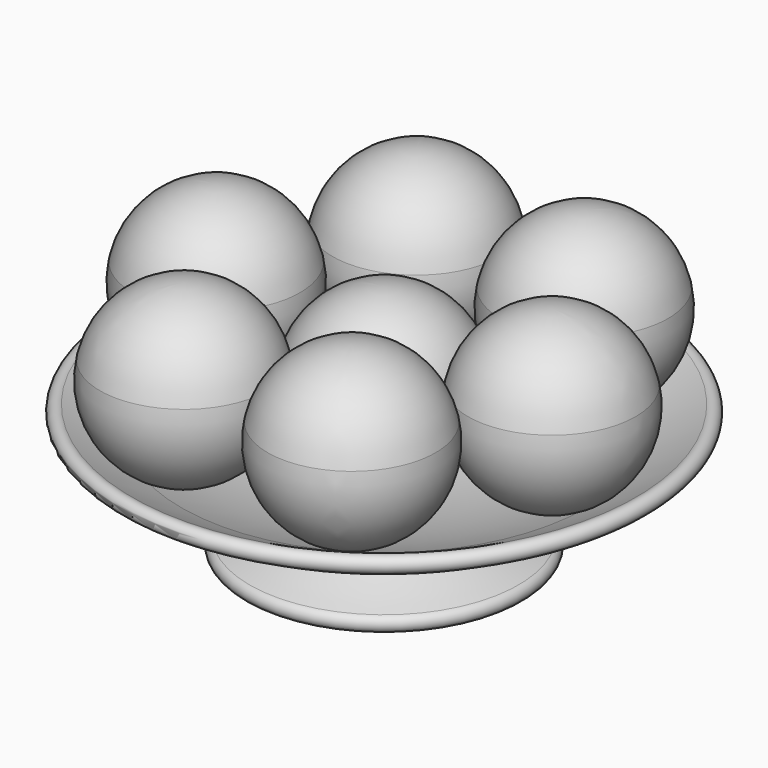
from build123d import *

# Parameters (mm, degrees)
F3_COUNT = 6


# Not quite as in the source:
# - ends of sketch curves that miss each other by under 0.0002 mm in the source are joined


with BuildPart() as f1:
    # F0 (on Front) → F1 (revolve)
    with BuildSketch(Plane.XZ):
        with BuildLine():
            Line((0, 0), (0, 6))
            ThreePointArc((0, 6), (-39.2492027787, 10.1203091704), (-76.7870949738, 22.3015864419))
            ThreePointArc((-76.7870949738, 22.3015864419), (-86.2691485264, 26.8374773841), (-95.484375, 31.8934883861))
            ThreePointArc((-95.484375, 31.8934883861), (-99.5889922478, 30.8201211382), (-98.515625, 26.7155038904))
            ThreePointArc((-98.515625, 26.7155038904), (-65.5508476643, 11.3479203208), (-30.3056435334, 2.3693483113))
            ThreePointArc((-30.3056435334, 2.3693483113), (-27.8017288025, -0.1720901245), (-29.4984382911, -3.3105093466))
            ThreePointArc((-29.4984382911, -3.3105093466), (-40.0930790369, -7.8980196489), (-50.9418468112, -11.8471842547))
            ThreePointArc((-50.9418468112, -11.8471842547), (-52.8483196071, -15.637350673), (-49.0581531888, -17.5438234688))
            ThreePointArc((-49.0581531888, -17.5438234688), (-33.5820797087, -11.7059923363), (-18.641323434, -4.6093082771))
            ThreePointArc((-18.641323434, -4.6093082771), (-9.6013626919, -1.1694213994), (0, 0))
        make_face()
    revolve(axis=Axis((0, 0, 30.1891714334), (0, 0, -1)))


with BuildPart() as f1b:
    # F0 (on Front) → F1, piece 2 (revolve)
    with BuildSketch(Plane.XZ):
        with BuildLine():
            ThreePointArc((0, 71), (-20.4560623568, 63.7546928877), (-31.7914813855, 45.2492007909))
            Line((-31.7914813855, 45.2492007909), (0, 38.5))
            Line((0, 38.5), (0, 71))
        make_face()
        with BuildLine():
            ThreePointArc((-31.7914813855, 45.2492007909), (-25.2546928877, 18.0439376432), (0, 6))
            Line((0, 6), (0, 38.5))
            Line((0, 38.5), (-31.7914813855, 45.2492007909))
        make_face()
    revolve(axis=Axis((0, 0, 30.1891714334), (0, 0, -1)))


with BuildPart() as f2_1:
    # F2: copy of F1b
    add(f1b.part.moved(Location((-63.5829625642, 0, 13.4984025559))))


with BuildPart() as f3_1:
    # F3: instance of F2_1
    add(f2_1.part.rotate(Axis((0, 0, 30.1891714334), (0, 0, -1)), 1 * 360 / F3_COUNT))


with BuildPart() as f3_2:
    # F3: instance of F2_1
    add(f2_1.part.rotate(Axis((0, 0, 30.1891714334), (0, 0, -1)), 2 * 360 / F3_COUNT))


with BuildPart() as f3_3:
    # F3: instance of F2_1
    add(f2_1.part.rotate(Axis((0, 0, 30.1891714334), (0, 0, -1)), 3 * 360 / F3_COUNT))


with BuildPart() as f3_4:
    # F3: instance of F2_1
    add(f2_1.part.rotate(Axis((0, 0, 30.1891714334), (0, 0, -1)), 4 * 360 / F3_COUNT))


with BuildPart() as f3_5:
    # F3: instance of F2_1
    add(f2_1.part.rotate(Axis((0, 0, 30.1891714334), (0, 0, -1)), 5 * 360 / F3_COUNT))


solid = Compound([f1.part, f1b.part, f2_1.part, f3_1.part, f3_2.part, f3_3.part, f3_4.part, f3_5.part])
